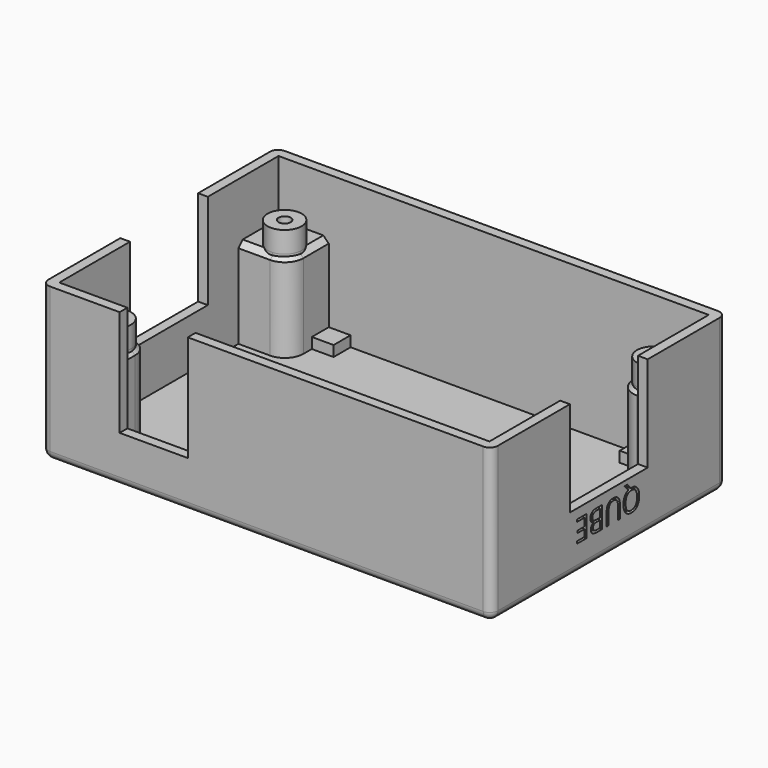
from build123d import *

# Parameters (mm, degrees)
F0_W          = 82.5
F0_H          = 53.85
F0_W_2        = 78.94
F0_H_2        = 50.29
F1_DEPTH      = 28.15
F2_W          = 82.5
F2_H          = 1.55
F3_DEPTH      = 53.85
F4_R          = 3.125
F4_R_2        = 1.125
F5_DEPTH      = 21.9
F7_DEPTH      = 18
F8_R          = 1.5
F9_T3_DEPTH   = 5.8401010127
F9_S4_R       = 3.125
F9_T5_DEPTH   = 5
F9_T8_DEPTH   = 5.8401010127
F9_S9_R       = 3.125
F9_T10_DEPTH  = 5
F9_T13_DEPTH  = 5.8401010127
F9_S14_R      = 3.125
F9_T15_DEPTH  = 5
F9_T18_DEPTH  = 5.8401010127
F9_S19_R      = 3.125
F9_T20_DEPTH  = 5
F9_T23_DEPTH  = 5.8401010127
F9_S24_R      = 3.125
F9_T25_DEPTH  = 5
F9_T28_DEPTH  = 5.8401010127
F9_S29_R      = 3.125
F9_T30_DEPTH  = 5
F9_T33_DEPTH  = 5.8401010127
F9_S34_R      = 3.125
F9_T35_DEPTH  = 5
F9_T38_DEPTH  = 5.8401010127
F9_S39_R      = 3.125
F9_T40_DEPTH  = 5
F9_T43_ANGLE  = 90
F9_S44_R      = 3.125
F9_T45_DEPTH  = 4
F9_T48_ANGLE  = 90
F9_S49_R      = 3.125
F9_T50_DEPTH  = 4
F9_T53_ANGLE  = 90
F9_S54_R      = 3.125
F9_T55_DEPTH  = 4
F9_T58_ANGLE  = 90
F9_S59_R      = 3.125
F9_T60_DEPTH  = 4
F10_DEPTH     = 7
F11_W         = 17.85
F11_H         = 17.5
F12_DEPTH     = 137.9
F13_W         = 12.5
F13_H         = 19.5
F14_DEPTH     = 25
F16_TEXT_SIZE = 5.5035833333
F17_DEPTH     = 0.85
F15_TEXT_SIZE = 5.5035773253
F18_DEPTH     = 0.85
F19_W         = 4.175
F19_H         = 2
F20_DEPTH     = 15
F21_W         = 4.175
F21_H         = 2
F22_DEPTH     = 15


# Not quite as in the source:
# - a fillet or chamfer that OpenCascade refuses, or shapes differently, is made with other operations: its cross-section is extruded or revolved along the edge and cut away or added
# - Text() gives the source's letters only with a copy of the font that has no kerning and outlines rounded to 1/6400 em; it was checked with that copy


with BuildPart() as f1:
    # F0 (on Top) → F1 (new body)
    with BuildSketch(Plane.XY):
        with Locations((41.25, 26.925)):
            Rectangle(F0_W, F0_H)
        with Locations((41.25, 26.925)):
            Rectangle(F0_W_2, F0_H_2, mode=Mode.SUBTRACT)
    extrude(amount=F1_DEPTH)

    # F2 (on Front) → F3 (join)
    with BuildSketch(Plane.XZ):
        with Locations((41.25, 0.775)):
            Rectangle(F2_W, F2_H)
    extrude(amount=-F3_DEPTH)

    # F4 (on Top) → F5 (join)
    with BuildSketch(Plane.XY):
        with Locations((7.36, 46.4899988616)):
            Circle(F4_R)
        with Locations((7.36, 46.4899988616)):
            Circle(F4_R_2, mode=Mode.SUBTRACT)
        with Locations((7.36, 7.36)):
            Circle(F4_R)
        with Locations((7.36, 7.36)):
            Circle(F4_R_2, mode=Mode.SUBTRACT)
        with Locations((75.1400032783, 7.36)):
            Circle(F4_R)
        with Locations((75.1400032783, 7.36)):
            Circle(F4_R_2, mode=Mode.SUBTRACT)
        with Locations((75.1400032783, 46.4899986982)):
            Circle(F4_R)
        with Locations((75.1400032783, 46.4899986982)):
            Circle(F4_R_2, mode=Mode.SUBTRACT)
    extrude(amount=F5_DEPTH)

    # F6 (on Top) → F7 (join)
    with BuildSketch(Plane.XY):
        with BuildLine():
            Line((0, 11), (0, 0))
            Line((0, 0), (11, 0))
            Line((11, 0), (11, 7.6201010127))
            ThreePointArc((11, 7.6201010127), (10.0100505063, 10.0100505063), (7.6201010127, 11))
            Line((7.6201010127, 11), (0, 11))
        make_face()
        with BuildLine():
            Line((0, 53.85), (0, 42.85))
            Line((0, 42.85), (7.6201010127, 42.85))
            ThreePointArc((7.6201010127, 42.85), (10.0100505063, 43.8399494937), (11, 46.2298989873))
            Line((11, 46.2298989873), (11, 53.85))
            Line((11, 53.85), (0, 53.85))
        make_face()
        with BuildLine():
            Line((71.5, 7.6201010127), (71.5, 0))
            Line((71.5, 0), (82.5, 0))
            Line((82.5, 0), (82.5, 11))
            Line((82.5, 11), (74.8798989873, 11))
            ThreePointArc((74.8798989873, 11), (72.4899494937, 10.0100505063), (71.5, 7.6201010127))
        make_face()
        with BuildLine():
            Line((74.8798989873, 42.85), (82.5, 42.85))
            Line((82.5, 42.85), (82.5, 53.85))
            Line((82.5, 53.85), (71.5, 53.85))
            Line((71.5, 53.85), (71.5, 46.2298989873))
            ThreePointArc((71.5, 46.2298989873), (72.4899494937, 43.8399494937), (74.8798989873, 42.85))
        make_face()
    extrude(amount=F7_DEPTH)

    # F8
    f8_edges = [f1.edges().sort_by_distance(p)[0] for p in [
        (41.25, 53.85, 0),
        (0, 26.925, 0),
        (41.25, 0, 0),
        (82.5, 26.925, 0),
        (82.5, 53.85, 14.075),
        (82.5, 0, 14.075),
        (0, 0, 14.075),
        (0, 53.85, 14.075),
    ]]
    fillet(f8_edges, radius=F8_R)

    # F9: chamfer of 1 on 12 edges, made by hand


with BuildPart() as f9_tool1:
    # F9_s2 → F9_t3 (new body)
    with BuildSketch(Plane.XZ.offset(-46.2298989873)):
        Polygon((10, 18), (11, 17), (11, 18), align=None)
    extrude(amount=-F9_T3_DEPTH)

    # F9_s4 → F9_t5 (cut, symmetric)
    with BuildSketch(Plane.XY.offset(17.5)):
        with Locations((7.36, 46.4899988616)):
            Circle(F9_S4_R)
    extrude(amount=F9_T5_DEPTH, both=True, mode=Mode.SUBTRACT)


with BuildPart() as f9_tool6:
    # F9_s7 → F9_t8 (new body)
    with BuildSketch(Plane.YZ.offset(1.78)):
        Polygon((42.85, 17), (43.85, 18), (42.85, 18), align=None)
    extrude(amount=F9_T8_DEPTH)

    # F9_s9 → F9_t10 (cut, symmetric)
    with BuildSketch(Plane.XY.offset(17.5)):
        with Locations((7.36, 46.4899988616)):
            Circle(F9_S9_R)
    extrude(amount=F9_T10_DEPTH, both=True, mode=Mode.SUBTRACT)


with BuildPart() as f9_tool11:
    # F9_s12 → F9_t13 (new body)
    with BuildSketch(Plane.YZ.offset(7.6201010127)):
        Polygon((10, 18), (11, 17), (11, 18), align=None)
    extrude(amount=-F9_T13_DEPTH)

    # F9_s14 → F9_t15 (cut, symmetric)
    with BuildSketch(Plane.XY.offset(17.5)):
        with Locations((7.36, 7.36)):
            Circle(F9_S14_R)
    extrude(amount=F9_T15_DEPTH, both=True, mode=Mode.SUBTRACT)


with BuildPart() as f9_tool16:
    # F9_s17 → F9_t18 (new body)
    with BuildSketch(Plane.XZ.offset(-1.78)):
        Polygon((11, 17), (10, 18), (11, 18), align=None)
    extrude(amount=-F9_T18_DEPTH)

    # F9_s19 → F9_t20 (cut, symmetric)
    with BuildSketch(Plane.XY.offset(17.5)):
        with Locations((7.36, 7.36)):
            Circle(F9_S19_R)
    extrude(amount=F9_T20_DEPTH, both=True, mode=Mode.SUBTRACT)


with BuildPart() as f9_tool21:
    # F9_s22 → F9_t23 (new body)
    with BuildSketch(Plane.XZ.offset(-7.6201010127)):
        Polygon((72.5, 18), (71.5, 17), (71.5, 18), align=None)
    extrude(amount=F9_T23_DEPTH)

    # F9_s24 → F9_t25 (cut, symmetric)
    with BuildSketch(Plane.XY.offset(17.5)):
        with Locations((75.1400032783, 7.36)):
            Circle(F9_S24_R)
    extrude(amount=F9_T25_DEPTH, both=True, mode=Mode.SUBTRACT)


with BuildPart() as f9_tool26:
    # F9_s27 → F9_t28 (new body)
    with BuildSketch(Plane.YZ.offset(80.72)):
        Polygon((10, 18), (11, 17), (11, 18), align=None)
    extrude(amount=-F9_T28_DEPTH)

    # F9_s29 → F9_t30 (cut, symmetric)
    with BuildSketch(Plane.XY.offset(17.5)):
        with Locations((75.1400032783, 7.36)):
            Circle(F9_S29_R)
    extrude(amount=F9_T30_DEPTH, both=True, mode=Mode.SUBTRACT)


with BuildPart() as f9_tool31:
    # F9_s32 → F9_t33 (new body)
    with BuildSketch(Plane.XZ.offset(-52.07)):
        Polygon((71.5, 17), (72.5, 18), (71.5, 18), align=None)
    extrude(amount=F9_T33_DEPTH)

    # F9_s34 → F9_t35 (cut, symmetric)
    with BuildSketch(Plane.XY.offset(17.5)):
        with Locations((75.1400032783, 46.4899986982)):
            Circle(F9_S34_R)
    extrude(amount=F9_T35_DEPTH, both=True, mode=Mode.SUBTRACT)


with BuildPart() as f9_tool36:
    # F9_s37 → F9_t38 (new body)
    with BuildSketch(Plane.YZ.offset(74.8798989873)):
        Polygon((43.85, 18), (42.85, 17), (42.85, 18), align=None)
    extrude(amount=F9_T38_DEPTH)

    # F9_s39 → F9_t40 (cut, symmetric)
    with BuildSketch(Plane.XY.offset(17.5)):
        with Locations((75.1400032783, 46.4899986982)):
            Circle(F9_S39_R)
    extrude(amount=F9_T40_DEPTH, both=True, mode=Mode.SUBTRACT)


with BuildPart() as f9_tool41:
    # F9_s42 → F9_t43 (revolve)
    with BuildSketch(Plane.XZ.offset(-7.6201010127)):
        Polygon((10, 18), (11, 17), (11, 18), align=None)
    revolve(axis=Axis((7.6201010127, 7.6201010127, 18), (0, 0, 1)), revolution_arc=F9_T43_ANGLE)

    # F9_s44 → F9_t45 (cut, symmetric)
    with BuildSketch(Plane.XY.offset(17.5)):
        with Locations((7.36, 7.36)):
            Circle(F9_S44_R)
    extrude(amount=F9_T45_DEPTH, both=True, mode=Mode.SUBTRACT)


with BuildPart() as f9_tool46:
    # F9_s47 → F9_t48 (revolve)
    with BuildSketch(Plane.YZ.offset(7.6201010127)):
        Polygon((43.85, 18), (42.85, 17), (42.85, 18), align=None)
    revolve(axis=Axis((7.6201010127, 46.2298989873, 18), (0, 0, 1)), revolution_arc=F9_T48_ANGLE)

    # F9_s49 → F9_t50 (cut, symmetric)
    with BuildSketch(Plane.XY.offset(17.5)):
        with Locations((7.36, 46.4899988616)):
            Circle(F9_S49_R)
    extrude(amount=F9_T50_DEPTH, both=True, mode=Mode.SUBTRACT)


with BuildPart() as f9_tool51:
    # F9_s52 → F9_t53 (revolve)
    with BuildSketch(Plane.XZ.offset(-46.2298989873)):
        Polygon((72.5, 18), (71.5, 17), (71.5, 18), align=None)
    revolve(axis=Axis((74.8798989873, 46.2298989873, 18), (0, 0, 1)), revolution_arc=F9_T53_ANGLE)

    # F9_s54 → F9_t55 (cut, symmetric)
    with BuildSketch(Plane.XY.offset(17.5)):
        with Locations((75.1400032783, 46.4899986982)):
            Circle(F9_S54_R)
    extrude(amount=F9_T55_DEPTH, both=True, mode=Mode.SUBTRACT)


with BuildPart() as f9_tool56:
    # F9_s57 → F9_t58 (revolve)
    with BuildSketch(Plane.YZ.offset(74.8798989873)):
        Polygon((10, 18), (11, 17), (11, 18), align=None)
    revolve(axis=Axis((74.8798989873, 7.6201010127, 18), (0, 0, 1)), revolution_arc=F9_T58_ANGLE)

    # F9_s59 → F9_t60 (cut, symmetric)
    with BuildSketch(Plane.XY.offset(17.5)):
        with Locations((75.1400032783, 7.36)):
            Circle(F9_S59_R)
    extrude(amount=F9_T60_DEPTH, both=True, mode=Mode.SUBTRACT)


with BuildPart() as f1_1:
    add(f1.part)

    # F9_t61: cut F9_tool1, F9_tool6, F9_tool11, F9_tool16, F9_tool21, F9_tool26, F9_tool31, F9_tool36, F9_tool41, F9_tool46, F9_tool51, F9_tool56
    add([f9_tool1.part, f9_tool6.part, f9_tool11.part, f9_tool16.part, f9_tool21.part, f9_tool26.part, f9_tool31.part, f9_tool36.part, f9_tool41.part, f9_tool46.part, f9_tool51.part, f9_tool56.part], mode=Mode.SUBTRACT)

    # F10 (cut): faces of the model
    f10_faces = [f1_1.faces().sort_by_distance(p)[0] for p in [
        (7.36, 7.36, 18),
        (7.36, 46.4899988616, 18),
        (75.1400032783, 46.4899986982, 18),
        (75.1400032783, 7.36, 18),
    ]]
    extrude(f10_faces, amount=-F10_DEPTH, mode=Mode.SUBTRACT)

    # F11 (on Right) → F12 (cut)
    with BuildSketch(Plane.YZ):
        with Locations((26.925, 19.4)):
            Rectangle(F11_W, F11_H)
    extrude(amount=F12_DEPTH, mode=Mode.SUBTRACT)

    # F13 (on Front) → F14 (cut)
    with BuildSketch(Plane.XZ):
        with Locations((20.53, 18.4)):
            Rectangle(F13_W, F13_H)
    extrude(amount=-F14_DEPTH, mode=Mode.SUBTRACT)

    # F16 (on face) → F17 (cut)
    with BuildSketch(Plane.YZ.offset(82.5)):
        with Locations(Location((34.240990267, 8.8747626887), (0, 0, 180))):
            Text('QUBE', F16_TEXT_SIZE, font='Open Sans', text_align=(TextAlign.LEFT, TextAlign.BOTTOM))
    extrude(amount=-F17_DEPTH, mode=Mode.SUBTRACT)

    # F15 (on face) → F18 (cut)
    with BuildSketch(Plane(origin=(0, 0, 0), x_dir=(0, -1, 0), z_dir=(-1, 0, 0))):
        with Locations(Location((-14.8002535105, 7.5747545177), (0, 0, -180))):
            Text('SCANNER', F15_TEXT_SIZE, font='Open Sans', text_align=(TextAlign.LEFT, TextAlign.BOTTOM))
    extrude(amount=-F18_DEPTH, mode=Mode.SUBTRACT)

    # F19 (on Right) → F20 (join)
    with BuildSketch(Plane.YZ):
        with Locations((50.2625, 2.4933788916)):
            Rectangle(F19_W, F19_H)
        with Locations((3.5875, 2.5)):
            Rectangle(F19_W, F19_H)
    extrude(amount=F20_DEPTH)

    # F21 (on face) → F22 (join)
    with BuildSketch(Plane.YZ.offset(82.5)):
        with Locations((3.5875, 2.5)):
            Rectangle(F21_W, F21_H)
        with Locations((50.2625, 2.5)):
            Rectangle(F21_W, F21_H)
    extrude(amount=-F22_DEPTH)


solid = f1_1.part
